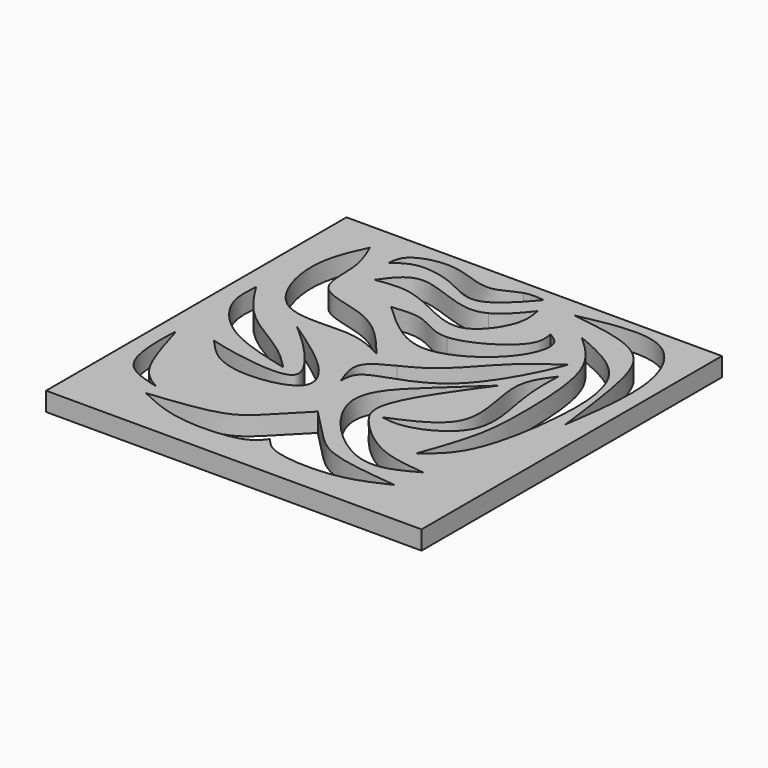
from build123d import *

# Parameters (mm, degrees)
F1_DEPTH = 5.08
F2_DEPTH = 5.08


with BuildPart() as f1:
    # F0 (on Top) → F1 (new body)
    with BuildSketch(Plane.XY):
        with BuildLine():
            add(Edge.make_bspline(
                [(0, 47.116682), (0, 48.344455), (0, 49.572227), (0, 50.8)],
                knots=[47.116682, 47.116682, 47.116682, 47.116682, 50.8, 50.8, 50.8, 50.8], degree=3))
            Line((0, 50.8), (-50.8, 50.8))
            Line((-50.8, 50.8), (-50.8, -50.8))
            Line((-50.8, -50.8), (0, -50.8))
            Line((0, -50.8), (0, -38.48964))
            add(Edge.make_bspline(
                [(-33.663414, -38.48964), (-29.732882, -40.337693), (-21.486909, -44.214775), (-3.657213, -43.251238), (-0.968234, -39.750254), (0, -38.48964)],
                knots=[0, 0, 0, 0, 0.368228, 0.772515, 1, 1, 1, 1], degree=3))
            add(Edge.make_bspline(
                [(0, -22.397682), (-2.786565, -25.294679), (-7.913403, -30.624695), (-14.206299, -36.43309), (-26.295468, -37.710873), (-33.663414, -38.48964)],
                knots=[0, 0, 0, 0, 0.31741, 0.583984, 1, 1, 1, 1], degree=3))
            Line((0, -22.397682), (0, -8.26285))
            Line((0, -8.26285), (0, -1.729301))
            add(Edge.make_bspline(
                [(-5.031325, -8.26285), (-4.976317, -6.533701), (-4.890437, -3.834029), (-1.496301, -2.294252), (0, -1.729301)],
                knots=[0, 0, 0, 0, 0.178027, 0.277948, 0.277948, 0.277948, 0.277948], degree=3))
            add(Edge.make_bspline(
                [(0, 4.455615), (-2.772212, 3.050297), (-8.346493, 0.137996), (-6.220023, -5.250633), (-5.031325, -8.26285)],
                knots=[0.637907, 0.637907, 0.637907, 0.637907, 0.797592, 1, 1, 1, 1], degree=3))
            add(Edge.make_bspline(
                [(0, 4.455615), (0, 7.698795), (0, 10.941974), (0, 14.185153)],
                knots=[4.455615, 4.455615, 4.455615, 4.455615, 14.185153, 14.185153, 14.185153, 14.185153], degree=3))
            add(Edge.make_bspline(
                [(0, 14.185153), (-4.610965, 14.057073), (-11.61146, 18.791704), (-15.886601, 22.84856), (-17.821625, 24.684787)],
                knots=[0.598896, 0.598896, 0.598896, 0.598896, 0.818451, 1, 1, 1, 1], degree=3))
            add(Edge.make_bspline(
                [(-17.821625, 24.684787), (-14.89535, 25.01102), (-8.823373, 25.68795), (-3.904245, 21.123598), (0, 21.264449)],
                knots=[0, 0, 0, 0, 0.229166, 0.475515, 0.475515, 0.475515, 0.475515], degree=3))
            add(Edge.make_bspline(
                [(0, 21.264449), (0, 23.067417), (0, 24.870386), (0, 26.673354)],
                knots=[21.264449, 21.264449, 21.264449, 21.264449, 26.673354, 26.673354, 26.673354, 26.673354], degree=3))
            add(Edge.make_bspline(
                [(0, 26.673354), (-3.549101, 25.56339), (-11.426009, 29.673997), (-20.088104, 33.408685), (-25.663836, 32.56426), (-28.321266, 32.161802)],
                knots=[0.39294, 0.39294, 0.39294, 0.39294, 0.6148, 0.816411, 1, 1, 1, 1], degree=3))
            add(Edge.make_bspline(
                [(-28.321266, 32.161802), (-26.212436, 35.150805), (-21.300029, 42.113526), (-7.101559, 32.957841), (-1.103708, 34.710754), (0, 35.267232)],
                knots=[0, 0, 0, 0, 0.284809, 0.663447, 0.756597, 0.756597, 0.756597, 0.756597], degree=3))
            add(Edge.make_bspline(
                [(0, 35.267232), (0, 37.356338), (0, 39.445444), (0, 41.53455)],
                knots=[35.267232, 35.267232, 35.267232, 35.267232, 41.53455, 41.53455, 41.53455, 41.53455], degree=3))
            add(Edge.make_bspline(
                [(-30.836448, 39.940536), (-29.349299, 41.158373), (-25.831723, 44.038945), (-14.304535, 41.940326), (-6.967066, 36.213576), (-1.436349, 40.259398), (0, 41.53455)],
                knots=[0, 0, 0, 0, 0.186015, 0.439984, 0.690005, 0.788118, 0.788118, 0.788118, 0.788118], degree=3))
            add(Edge.make_bspline(
                [(0, 47.116682), (-2.203233, 46.423428), (-7.383268, 42.302808), (-18.393291, 48.944751), (-30.365356, 45.375787), (-30.703046, 41.479704), (-30.836448, 39.940536)],
                knots=[0.166165, 0.166165, 0.166165, 0.166165, 0.364283, 0.612254, 0.846819, 1, 1, 1, 1], degree=3))
        make_face()
        with BuildLine():
            add(Edge.make_bspline(
                [(-33.953361, -34.720354), (-36.404982, -33.252861), (-41.951104, -29.93295), (-45.987374, -12.527915), (-46.327003, -12.743329), (-46.348516, -12.757003)],
                knots=[0, 0, 0, 0, 0.425967, 0.963631, 1, 1, 1, 1], degree=3))
            add(Edge.make_bspline(
                [(-46.348516, -12.757003), (-46.469725, -15.599171), (-46.715789, -21.369012), (-44.789983, -31.788585), (-37.634331, -33.724496), (-33.953361, -34.720354)],
                knots=[0, 0, 0, 0, 0.320377, 0.650392, 1, 1, 1, 1], degree=3))
        make_face(mode=Mode.SUBTRACT)
        with BuildLine():
            add(Edge.make_bspline(
                [(-43.449067, -12.757003), (-41.198987, -15.675043), (-36.201672, -22.155862), (-16.180181, -28.872506), (-5.696461, -15.518769), (0, -8.26285)],
                knots=[0, 0, 0, 0, 0.272199, 0.60454, 1, 1, 1, 1], degree=3))
            add(Edge.make_bspline(
                [(0, -8.26285), (-0.687741, -11.81785), (-2.216072, -19.717937), (-13.756187, -34.230048), (-26.430737, -35.219982), (-38.927173, -28.709158), (-41.879988, -18.292349), (-43.449067, -12.757003)],
                knots=[0, 0, 0, 0, 0.183479, 0.407735, 0.591656, 0.783012, 1, 1, 1, 1], degree=3))
        make_face(mode=Mode.SUBTRACT)
        with BuildLine():
            add(Edge.make_bspline(
                [(-27.605377, 5.11729), (-24.612769, 2.485721), (-19.012967, -2.438501), (-9.744661, -15.281479), (-29.650876, -12.82008), (-35.06647, -11.359554), (-37.468672, -10.711707)],
                knots=[0, 0, 0, 0, 0.264716, 0.49534, 0.776148, 1, 1, 1, 1], degree=3))
            add(Edge.make_bspline(
                [(-37.468672, -10.711707), (-35.456306, -12.983771), (-31.133077, -17.864919), (-19.194065, -19.285743), (-7.594141, -15.639977), (-10.870913, -6.172995), (-21.096612, 0.726007), (-27.605377, 5.11729)],
                knots=[0, 0, 0, 0, 0.179329, 0.385258, 0.572661, 0.727995, 1, 1, 1, 1], degree=3))
        make_face(mode=Mode.SUBTRACT)
        with BuildLine():
            add(Edge.make_bspline(
                [(-45.820653, 14.026068), (-46.029645, 11.288099), (-46.50178, 5.102723), (-37.167317, -6.445303), (-25.030719, -9.458069), (-18.378429, -11.109419)],
                knots=[0, 0, 0, 0, 0.264105, 0.596643, 1, 1, 1, 1], degree=3))
            add(Edge.make_bspline(
                [(-18.378429, -11.109419), (-20.353704, -9.082091), (-24.850653, -4.466637), (-38.44457, 2.34861), (-43.392811, 10.182428), (-45.820653, 14.026068)],
                knots=[0, 0, 0, 0, 0.285196, 0.649284, 1, 1, 1, 1], degree=3))
        make_face(mode=Mode.SUBTRACT)
        with BuildLine():
            add(Edge.make_bspline(
                [(-38.264096, 43.059148), (-40.299736, 38.737966), (-44.630781, 29.544179), (-37.679929, 6.88301), (-16.989211, 11.227092), (-10.001158, 7.647786), (-6.924279, 6.071799)],
                knots=[0, 0, 0, 0, 0.24491, 0.521072, 0.789125, 1, 1, 1, 1], degree=3))
            add(Edge.make_bspline(
                [(-38.264096, 43.059148), (-37.011136, 40.172238), (-34.43687, 34.240943), (-36.362298, 20.409505), (-17.915188, 19.672077), (-10.6901, 10.731668), (-6.924279, 6.071799)],
                knots=[0, 0, 0, 0, 0.216483, 0.444774, 0.710608, 1, 1, 1, 1], degree=3))
        make_face(mode=Mode.SUBTRACT)
        with BuildLine():
            add(Edge.make_bspline(
                [(0, -8.26285), (-0.687741, -11.81785), (-2.216072, -19.717937), (-13.756187, -34.230048), (-26.430737, -35.219982), (-38.927173, -28.709158), (-41.879988, -18.292349), (-43.449067, -12.757003)],
                knots=[0, 0, 0, 0, 0.183479, 0.407735, 0.591656, 0.783012, 1, 1, 1, 1], degree=3))
            add(Edge.make_bspline(
                [(-43.449067, -12.757003), (-41.198987, -15.675043), (-36.201672, -22.155862), (-16.180181, -28.872506), (-5.696461, -15.518769), (0, -8.26285)],
                knots=[0, 0, 0, 0, 0.272199, 0.60454, 1, 1, 1, 1], degree=3))
        make_face()
    extrude(amount=F1_DEPTH)

    # F0 (on Top) → F2 (join)
    with BuildSketch(Plane.XY):
        with BuildLine():
            Line((50.8, -50.8), (50.8, 50.8))
            Line((50.8, 50.8), (0, 50.8))
            add(Edge.make_bspline(
                [(0, 47.116682), (0, 48.344455), (0, 49.572227), (0, 50.8)],
                knots=[47.116682, 47.116682, 47.116682, 47.116682, 50.8, 50.8, 50.8, 50.8], degree=3))
            add(Edge.make_bspline(
                [(5.4067, 47.261655), (3.62729, 47.479889), (1.847881, 47.698124), (0, 47.116682)],
                knots=[0, 0, 0, 0, 0.166165, 0.166165, 0.166165, 0.166165], degree=3))
            add(Edge.make_bspline(
                [(0, 41.53455), (2.594549, 43.837922), (5.219133, 47.118052), (5.380365, 47.241512), (5.4067, 47.261655)],
                knots=[0.788118, 0.788118, 0.788118, 0.788118, 0.965345, 1, 1, 1, 1], degree=3))
            add(Edge.make_bspline(
                [(0, 35.267232), (0, 37.356338), (0, 39.445444), (0, 41.53455)],
                knots=[35.267232, 35.267232, 35.267232, 35.267232, 41.53455, 41.53455, 41.53455, 41.53455], degree=3))
            add(Edge.make_bspline(
                [(0, 35.267232), (2.883992, 36.721313), (5.21824, 39.611833), (7.55249, 42.502351)],
                knots=[0.756597, 0.756597, 0.756597, 0.756597, 1, 1, 1, 1], degree=3))
            add(Edge.make_bspline(
                [(7.55249, 42.502351), (7.936335, 40.404925), (8.823035, 35.559773), (3.564782, 27.788222), (0, 26.673354)],
                knots=[0, 0, 0, 0, 0.170101, 0.39294, 0.39294, 0.39294, 0.39294], degree=3))
            add(Edge.make_bspline(
                [(0, 21.264449), (0, 23.067417), (0, 24.870386), (0, 26.673354)],
                knots=[21.264449, 21.264449, 21.264449, 21.264449, 26.673354, 26.673354, 26.673354, 26.673354], degree=3))
            add(Edge.make_bspline(
                [(0, 21.264449), (5.236034, 21.453345), (17.419432, 28.907082), (16.603967, 34.069379), (16.302183, 35.979848)],
                knots=[0.475515, 0.475515, 0.475515, 0.475515, 0.805898, 1, 1, 1, 1], degree=3))
            add(Edge.make_bspline(
                [(16.302183, 35.979848), (17.683335, 35.146634), (21.111836, 33.078304), (17.465945, 21.689868), (5.65155, 14.342137), (0, 14.185153)],
                knots=[0, 0, 0, 0, 0.132855, 0.329793, 0.598896, 0.598896, 0.598896, 0.598896], degree=3))
            add(Edge.make_bspline(
                [(0, 4.455615), (0, 7.698795), (0, 10.941974), (0, 14.185153)],
                knots=[4.455615, 4.455615, 4.455615, 4.455615, 14.185153, 14.185153, 14.185153, 14.185153], degree=3))
            add(Edge.make_bspline(
                [(27.442537, 27.110461), (24.03591, 24.708326), (16.727222, 19.554709), (8.875386, 8.898118), (1.702751, 5.318792), (0, 4.455615)],
                knots=[0, 0, 0, 0, 0.251616, 0.539825, 0.637907, 0.637907, 0.637907, 0.637907], degree=3))
            add(Edge.make_bspline(
                [(0, -1.729301), (3.948195, -0.238602), (18.750202, 3.720207), (28.892229, 29.030977), (27.603567, 27.323799), (27.442537, 27.110461)],
                knots=[0.277948, 0.277948, 0.277948, 0.277948, 0.541605, 0.942722, 1, 1, 1, 1], degree=3))
            Line((0, -1.729301), (0, -8.26285))
            Line((0, -8.26285), (0, -22.397682))
            add(Edge.make_bspline(
                [(0, -22.397682), (2.786565, -25.294679), (7.913403, -30.624695), (14.206299, -36.43309), (26.295468, -37.710873), (33.663414, -38.48964)],
                knots=[0, 0, 0, 0, 0.31741, 0.583984, 1, 1, 1, 1], degree=3))
            add(Edge.make_bspline(
                [(33.663414, -38.48964), (29.732882, -40.337693), (21.486909, -44.214775), (3.657213, -43.251238), (0.968234, -39.750254), (0, -38.48964)],
                knots=[0, 0, 0, 0, 0.368228, 0.772515, 1, 1, 1, 1], degree=3))
            Line((0, -38.48964), (0, -50.8))
            Line((0, -50.8), (50.8, -50.8))
        make_face()
        with BuildLine():
            add(Edge.make_bspline(
                [(27.949937, -45.810752), (28.041482, -45.833192), (28.133026, -45.855632), (28.224566, -45.878029)],
                knots=[0, 0, 0, 0, 0.007578, 0.007578, 0.007578, 0.007578], degree=3))
            add(Edge.make_bspline(
                [(28.224566, -45.878029), (28.094513, -45.877852), (28.000737, -45.855796), (27.949937, -45.810752)],
                knots=[0.899724, 0.899724, 0.899724, 0.899724, 0.931426, 0.931426, 0.931426, 0.931426], degree=3))
        make_face(mode=Mode.SUBTRACT)
        with BuildLine():
            add(Edge.make_bspline(
                [(44.476815, -19.788176), (43.873934, -23.776972), (42.623495, -32.050168), (35.390192, -43.444307), (29.042075, -45.879146), (28.224566, -45.878029)],
                knots=[0, 0, 0, 0, 0.337707, 0.70044, 0.899724, 0.899724, 0.899724, 0.899724], degree=3))
            add(Edge.make_bspline(
                [(28.224566, -45.878029), (31.769217, -46.745317), (39.777568, -48.564233), (49.365751, -31.820736), (46.038284, -23.631234), (44.476815, -19.788176)],
                knots=[0.007578, 0.007578, 0.007578, 0.007578, 0.301011, 0.671988, 1, 1, 1, 1], degree=3))
        make_face(mode=Mode.SUBTRACT)
        with BuildLine():
            add(Edge.make_bspline(
                [(22.513464, 10.87353), (18.734451, 7.400114), (11.122761, 0.40396), (-4.011428, -14.03931), (20.026913, -38.462349), (30.338214, -32.699529), (34.763657, -30.226201)],
                knots=[0, 0, 0, 0, 0.235072, 0.473482, 0.774027, 1, 1, 1, 1], degree=3))
            add(Edge.make_bspline(
                [(34.763657, -30.226201), (30.310577, -29.761409), (21.50513, -28.842338), (11.37318, -20.189427), (6.146005, -11.722265), (16.059198, 1.963211), (22.513464, 10.87353)],
                knots=[0, 0, 0, 0, 0.239672, 0.473923, 0.657483, 1, 1, 1, 1], degree=3))
        make_face(mode=Mode.SUBTRACT)
        with BuildLine():
            add(Edge.make_bspline(
                [(29.689603, 21.891449), (27.708938, 19.264221), (23.066274, 13.106019), (31.375447, -7.93973), (18.580491, -13.287933), (12.220412, -15.946403)],
                knots=[0, 0, 0, 0, 0.272304, 0.638279, 1, 1, 1, 1], degree=3))
            add(Edge.make_bspline(
                [(12.220412, -15.946403), (14.303682, -16.26309), (19.317712, -17.025294), (33.741595, -9.527025), (30.755215, 5.546052), (29.46114, 13.759807), (29.614579, 19.221147), (29.689603, 21.891449)],
                knots=[0, 0, 0, 0, 0.167066, 0.402095, 0.635914, 0.821982, 1, 1, 1, 1], degree=3))
        make_face(mode=Mode.SUBTRACT)
        with BuildLine():
            add(Edge.make_bspline(
                [(22.440977, 38.853243), (25.795104, 35.7975), (33.378263, 28.888936), (34.269727, 5.551143), (33.762186, -8.998172), (30.096887, -19.142667), (28.239883, -24.282321)],
                knots=[0, 0, 0, 0, 0.229177, 0.518134, 0.755865, 1, 1, 1, 1], degree=3))
            add(Edge.make_bspline(
                [(28.239883, -24.282321), (30.70946, -22.392221), (36.800254, -17.730608), (41.609891, 2.910262), (42.182358, 30.504507), (28.707442, 36.203118), (22.440977, 38.853243)],
                knots=[0, 0, 0, 0, 0.182822, 0.450899, 0.744642, 1, 1, 1, 1], degree=3))
        make_face(mode=Mode.SUBTRACT)
        with BuildLine():
            add(Edge.make_bspline(
                [(44.549294, 5.727004), (43.701212, 12.505502), (42.110435, 25.220195), (37.7023, 42.758286), (22.77267, 44.738955), (14.684945, 45.811929)],
                knots=[0, 0, 0, 0, 0.343532, 0.644377, 1, 1, 1, 1], degree=3))
            add(Edge.make_bspline(
                [(14.684945, 45.811929), (22.759032, 47.491197), (37.810058, 50.621545), (48.550233, 32.820192), (45.994705, 15.514897), (44.549294, 5.727004)],
                knots=[0, 0, 0, 0, 0.334536, 0.623613, 1, 1, 1, 1], degree=3))
        make_face(mode=Mode.SUBTRACT)
        with BuildLine():
            add(Edge.make_bspline(
                [(28.224566, -45.878029), (31.769217, -46.745317), (39.777568, -48.564233), (49.365751, -31.820736), (46.038284, -23.631234), (44.476815, -19.788176)],
                knots=[0.007578, 0.007578, 0.007578, 0.007578, 0.301011, 0.671988, 1, 1, 1, 1], degree=3))
            add(Edge.make_bspline(
                [(44.476815, -19.788176), (43.873934, -23.776972), (42.623495, -32.050168), (35.390192, -43.444307), (29.042075, -45.879146), (28.224566, -45.878029)],
                knots=[0, 0, 0, 0, 0.337707, 0.70044, 0.899724, 0.899724, 0.899724, 0.899724], degree=3))
        make_face()
    extrude(amount=F2_DEPTH)


solid = f1.part
